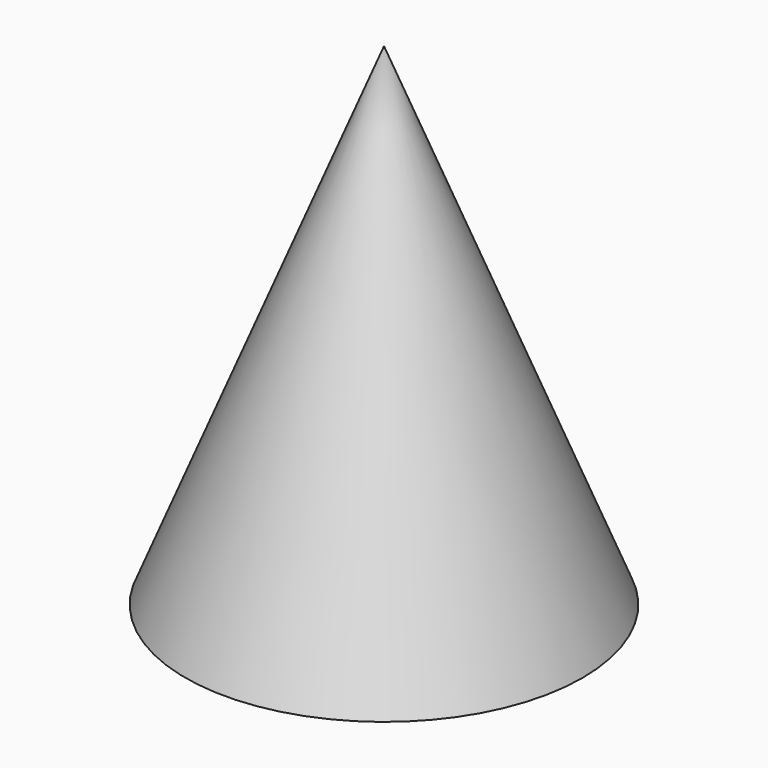
from build123d import *

# Parameters (mm, degrees)
F0_R     = 4.1008197162
F1_DEPTH = 12
F1_TAPER = 22
F2_R     = 2.5
F3_DEPTH = 2


with BuildPart() as f1:
    # F0 (on Top) → F1 (new body)
    with BuildSketch(Plane.XY):
        Circle(F0_R)
    extrude(amount=F1_DEPTH, taper=F1_TAPER)

    # F2 (on face) → F3 (cut)
    with BuildSketch(Plane(origin=(0, 0, 0), x_dir=(1, 0, 0), z_dir=(0, 0, -1))):
        Circle(F2_R)
    extrude(amount=-F3_DEPTH, mode=Mode.SUBTRACT)


solid = f1.part
